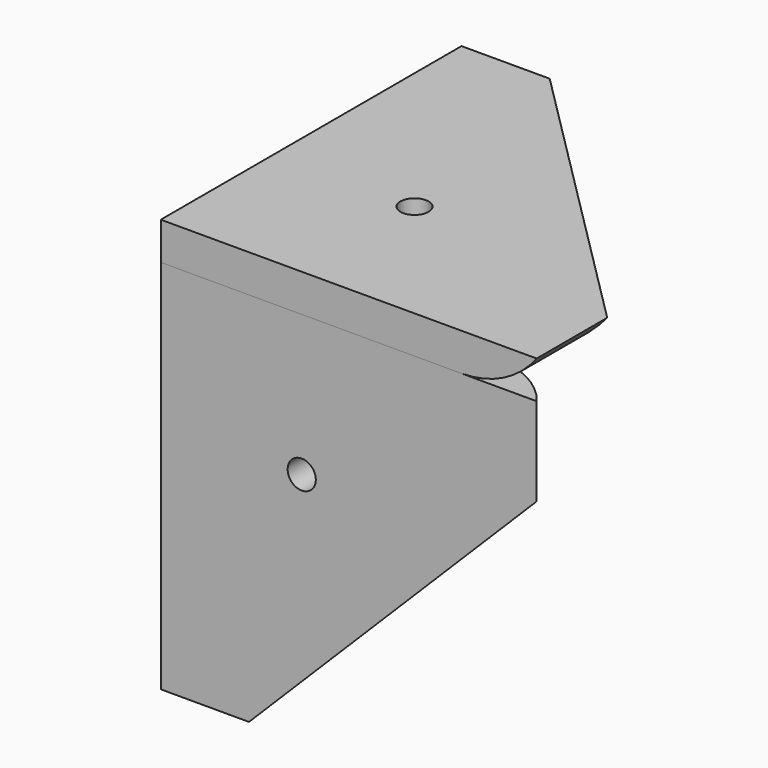
from build123d import *

# Parameters (mm, degrees)
F0_R          = 1.5
F1_DEPTH      = 4
F2_ANGLE      = 90
F3_ANGLE      = 90
F4_T1_DEPTH   = 83.2928317533
F4_T3_DEPTH   = 49.3873450905
F4_T5_DEPTH   = 49.3873450905
F4_2_T1_DEPTH = 83.2928317533
F4_2_T3_DEPTH = 49.3873450905
F4_2_T5_DEPTH = 49.3873450905
F4_3_T1_DEPTH = 83.2928317533
F4_3_T3_DEPTH = 49.3873450905
F4_3_T5_DEPTH = 49.3873450905


# Not quite as in the source:
# - a fillet or chamfer that OpenCascade refuses, or shapes differently, is made with other operations: its cross-section is extruded or revolved along the edge and cut away or added


with BuildPart() as f1:
    # F0 (on Front) → F1 (new body)
    with BuildSketch(Plane.XZ):
        Polygon((40, 0), (0, 0), (0, -40), (9.3873450905, -40), (40, -9.3873450905), align=None)
        with Locations((15, -15)):
            Circle(F0_R, mode=Mode.SUBTRACT)
    extrude(amount=-F1_DEPTH)


with BuildPart() as f2_1:
    # F2: copy of F1
    add(f1.part.rotate(Axis((20, 0, 0), (1, 0, 0)), F2_ANGLE))


with BuildPart() as f3_1:
    # F3: copy of F2_1
    add(f2_1.part.rotate(Axis((0, 20, 0), (0, 1, 0)), F3_ANGLE))

    # F4#3: fillet of radius 10 on 3 edges, made by hand

    # F4_3_s2 → F4_3_t1 (cut)
    with BuildSketch(Plane(origin=(0, 29.4484630785, 29.4484630785), x_dir=(1, 0, 0), z_dir=(0, -0.7071067812, -0.7071067812))):
        with BuildLine():
            ThreePointArc((0, -34.9221266183), (2.94427191, -31.3942625733), (4, -26.9221266183))
            Line((4, -26.9221266183), (4, -34.9221266183))
            Line((4, -34.9221266183), (0, -34.9221266183))
        make_face()
    extrude(amount=F4_3_T1_DEPTH, mode=Mode.SUBTRACT)

    # F4_3_s4 → F4_3_t3 (cut)
    with BuildSketch(Plane.XZ.offset(-29.3873450905)):
        with BuildLine():
            ThreePointArc((0, -40), (2.94427191, -36.472135955), (4, -32))
            Line((4, -32), (4, -40))
            Line((4, -40), (0, -40))
        make_face()
    extrude(amount=F4_3_T3_DEPTH, mode=Mode.SUBTRACT)

    # F4_3_s6 → F4_3_t5 (cut)
    with BuildSketch(Plane.XY.offset(-29.3873450905)):
        with BuildLine():
            ThreePointArc((0, 40), (2.94427191, 36.472135955), (4, 32))
            Line((4, 32), (4, 40))
            Line((4, 40), (0, 40))
        make_face()
    extrude(amount=F4_3_T5_DEPTH, mode=Mode.SUBTRACT)


with BuildPart() as f1_1:
    add(f1.part)

    # F4: fillet of radius 10 on 3 edges, made by hand

    # F4_s2 → F4_t1 (cut)
    with BuildSketch(Plane(origin=(-29.4484630785, 0, -29.4484630785), x_dir=(0, 1, 0), z_dir=(0.7071067812, 0, 0.7071067812))):
        with BuildLine():
            ThreePointArc((0, -34.9221266183), (2.94427191, -31.3942625733), (4, -26.9221266183))
            Line((4, -26.9221266183), (4, -34.9221266183))
            Line((4, -34.9221266183), (0, -34.9221266183))
        make_face()
    extrude(amount=F4_T1_DEPTH, mode=Mode.SUBTRACT)

    # F4_s4 → F4_t3 (cut)
    with BuildSketch(Plane.YZ.offset(-20)):
        with BuildLine():
            ThreePointArc((0, -40), (2.94427191, -36.472135955), (4, -32))
            Line((4, -32), (4, -40))
            Line((4, -40), (0, -40))
        make_face()
    extrude(amount=F4_T3_DEPTH, mode=Mode.SUBTRACT)

    # F4_s6 → F4_t5 (cut)
    with BuildSketch(Plane.XY.offset(-29.3873450905)):
        with BuildLine():
            ThreePointArc((40, 0), (36.472135955, 2.94427191), (32, 4))
            Line((32, 4), (40, 4))
            Line((40, 4), (40, 0))
        make_face()
    extrude(amount=F4_T5_DEPTH, mode=Mode.SUBTRACT)


with BuildPart() as f2_1_1:
    add(f2_1.part)

    # F4#2: fillet of radius 10 on 3 edges, made by hand

    # F4_2_s2 → F4_2_t1 (cut)
    with BuildSketch(Plane(origin=(-29.4484630785, 29.4484630785, 0), x_dir=(0, 0, 1), z_dir=(0.7071067812, -0.7071067812, 0))):
        with BuildLine():
            ThreePointArc((4, -34.9221266183), (1.05572809, -31.3942625733), (0, -26.9221266183))
            Line((0, -26.9221266183), (0, -34.9221266183))
            Line((0, -34.9221266183), (4, -34.9221266183))
        make_face()
    extrude(amount=F4_2_T1_DEPTH, mode=Mode.SUBTRACT)

    # F4_2_s4 → F4_2_t3 (cut)
    with BuildSketch(Plane.YZ.offset(-20)):
        with BuildLine():
            ThreePointArc((40, 4), (36.472135955, 1.05572809), (32, 0))
            Line((32, 0), (40, 0))
            Line((40, 0), (40, 4))
        make_face()
    extrude(amount=F4_2_T3_DEPTH, mode=Mode.SUBTRACT)

    # F4_2_s6 → F4_2_t5 (cut)
    with BuildSketch(Plane.XZ.offset(-29.3873450905)):
        with BuildLine():
            ThreePointArc((40, 4), (36.472135955, 1.05572809), (32, 0))
            Line((32, 0), (40, 0))
            Line((40, 0), (40, 4))
        make_face()
    extrude(amount=F4_2_T5_DEPTH, mode=Mode.SUBTRACT)


solid = Compound([f3_1.part, f1_1.part, f2_1_1.part])
